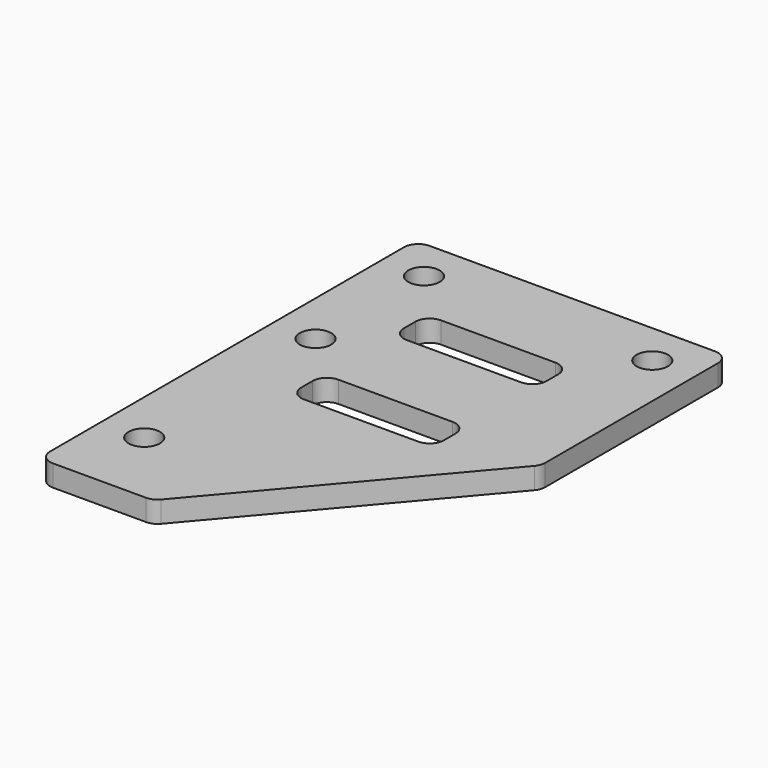
from build123d import *

# Parameters (mm, degrees)
F0_W     = 22
F0_H     = 33
F0_R     = 1.1
F1_DEPTH = 1.5
F2_R     = 1.1
F3_DEPTH = 1.5
F4_R     = 1


# Not quite as in the source:
# - a feature names something its author has since deleted; it is built from what else it names


with BuildPart() as f1:
    # F0 (on Top) → F1 (new body)
    with BuildSketch(Plane.XY):
        Rectangle(F0_W, F0_H)
        with Locations((-8, 13.5)):
            Circle(F0_R, mode=Mode.SUBTRACT)
        with Locations((8, 13.5)):
            Circle(F0_R, mode=Mode.SUBTRACT)
    extrude(amount=F1_DEPTH)

    # F2 (on face) → F3 (cut, through all)
    with BuildSketch(Plane.XY.offset(1.5)):
        with BuildLine():
            Line((4, 10), (-4, 10))
            ThreePointArc((-4, 10), (-4.7071067812, 9.7071067812), (-5, 9))
            Line((-5, 9), (-5, 8))
            ThreePointArc((-5, 8), (-4.7071067812, 7.2928932188), (-4, 7))
            Line((-4, 7), (4, 7))
            ThreePointArc((4, 7), (4.7071067812, 7.2928932188), (5, 8))
            Line((5, 8), (5, 9))
            ThreePointArc((5, 9), (4.7071067812, 9.7071067812), (4, 10))
        make_face()
        with BuildLine():
            Line((4, 1), (-4, 1))
            ThreePointArc((-4, 1), (-4.7071067812, 0.7071067812), (-5, 0))
            Line((-5, 0), (-5, -1))
            ThreePointArc((-5, -1), (-4.7071067812, -1.7071067812), (-4, -2))
            Line((-4, -2), (4, -2))
            ThreePointArc((4, -2), (4.7071067812, -1.7071067812), (5, -1))
            Line((5, -1), (5, 0))
            ThreePointArc((5, 0), (4.7071067812, 0.7071067812), (4, 1))
        make_face()
        Polygon((11, -16.5), (11, 0), (-3, -16.5), align=None)
        with Locations((-8, 4)):
            Circle(F2_R)
        with Locations((-8, -11)):
            Circle(F2_R)
    extrude(amount=-F3_DEPTH, mode=Mode.SUBTRACT)

    # F4
    f4_edges = [f1.edges().sort_by_distance(p)[0] for p in [
        (-11, 16.5, 0.75),
        (11, 16.5, 0.75),
        (-11, -16.5, 0.75),
        (11, 0, 0.75),
        (-3, -16.5, 0.75),
    ]]
    fillet(f4_edges, radius=F4_R)


solid = f1.part
